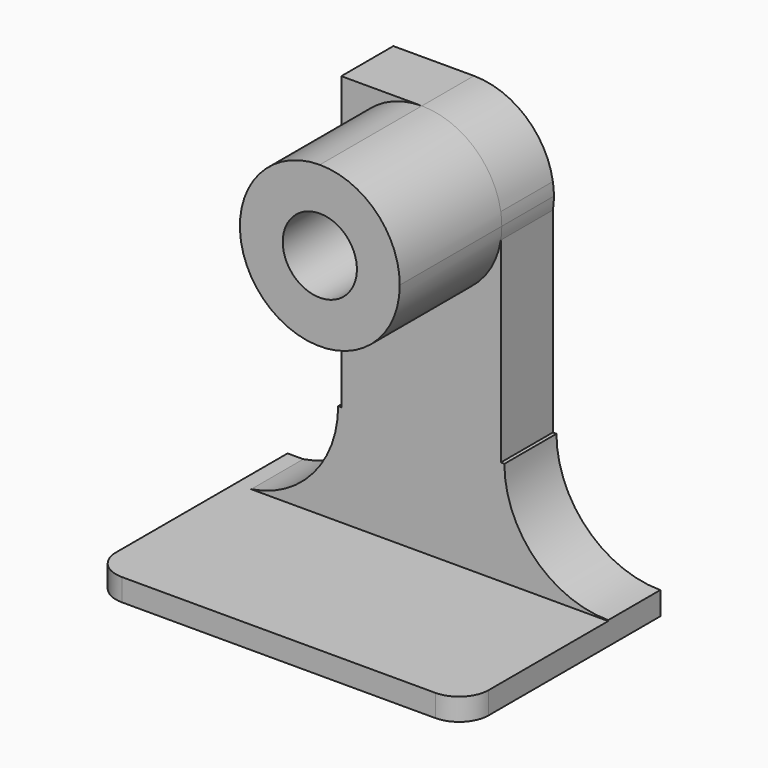
from build123d import *

# Parameters (mm, degrees)
F0_W      = 63.8407319784
F0_H      = 41.8170765042
F1_DEPTH  = 3.81
F2_R      = 5.08
F3_W      = 63.8407319784
F3_H      = 11.1512206495
F4_DEPTH  = 67.31
F6_DEPTH  = 21.844
F8_D      = 12.7
F9_W      = 18.1207312271
F9_H      = 49.9326833737
F10_DEPTH = 25.4
F12_DEPTH = 25.4


# Not quite as in the source:
# - a feature of the source that left no trace in its solid (it failed there, or was rolled back) is left out


with BuildPart() as f1:
    # F0 (on Top) → F1 (new body)
    with BuildSketch(Plane.XY):
        Rectangle(F0_W, F0_H)
    extrude(amount=F1_DEPTH)

    # F2
    f2_edges = [f1.edges().sort_by_distance(p)[0] for p in [
        (-31.920366, -20.908538, 1.905),
        (31.920366, -20.908538, 1.905),
    ]]
    fillet(f2_edges, radius=F2_R)

    # F3 (on face) → F4 (join)
    with BuildSketch(Plane.XY.offset(3.81)):
        with Locations((0, 15.3329279274)):
            Rectangle(F3_W, F3_H)
    extrude(amount=F4_DEPTH)

    # F5 (on face) → F6 (join)
    with BuildSketch(Plane.XZ.offset(-9.7573176026)):
        with BuildLine():
            ThreePointArc((1.435e-07, 71.12), (-9.6811538885, 47.7476271561), (13.6912190568, 57.4287809432))
            ThreePointArc((13.6912190568, 57.4287809432), (9.6811538885, 67.1099347302), (1.435e-07, 71.12))
        make_face()
    extrude(amount=F6_DEPTH)

    # F8 (through all)
    with Locations(Plane.XZ.offset(12.0866823974)):
        with Locations((0, 57.4287809432)):
            Hole(F8_D / 2)

    # F9 (on face) → F10 (cut)
    with BuildSketch(Plane.XZ.offset(-9.7573176026)):
        with Locations((-22.8600003757, 46.1536583132)):
            Rectangle(F9_W, F9_H)
        with BuildLine():
            Line((13.5208535939, 71.12), (-1.606e-07, 71.12))
            ThreePointArc((-1.606e-07, 71.12), (8.8873621455, 67.8433991962), (13.5208535939, 59.5819175746))
            Line((13.5208535939, 59.5819175746), (13.5208535939, 71.12))
        make_face()
        with BuildLine():
            Line((31.9203659892, 71.12), (13.5208535939, 71.12))
            Line((13.5208535939, 71.12), (13.5208535939, 59.5819175746))
            ThreePointArc((13.5208535939, 59.5819175746), (13.6485612365, 58.5087140134), (13.6912190568, 57.4287809432))
            ThreePointArc((13.6912190568, 57.4287809432), (13.6485612365, 56.3488478729), (13.5208535939, 55.2756443117))
            Line((13.5208535939, 55.2756443117), (13.5208535939, 21.7448789626))
            Line((13.5208535939, 21.7448789626), (31.9203659892, 21.7448789626))
            Line((31.9203659892, 21.7448789626), (31.9203659892, 71.12))
        make_face()
    extrude(amount=-F10_DEPTH, mode=Mode.SUBTRACT)

    # F11 (on face) → F12 (cut)
    with BuildSketch(Plane.XZ.offset(-9.7573176026)):
        with BuildLine():
            ThreePointArc((-29.2383271601, 3.81), (-18.5726517534, 9.7416628621), (-14.3372927251, 21.1873166263))
            Line((-14.3372927251, 21.1873166263), (-31.9203659892, 21.1873166263))
            Line((-31.9203659892, 21.1873166263), (-31.9203659892, 3.81))
            Line((-31.9203659892, 3.81), (-29.2383271601, 3.81))
        make_face()
        with BuildLine():
            ThreePointArc((14.1373165346, 21.7448789626), (19.3458511297, 9.1703641031), (31.9203659892, 3.9618295081))
            Line((31.9203659892, 3.9618295081), (31.9203659892, 21.7448789626))
            Line((31.9203659892, 21.7448789626), (14.1373165346, 21.7448789626))
        make_face()
    extrude(amount=-F12_DEPTH, mode=Mode.SUBTRACT)


solid = f1.part
